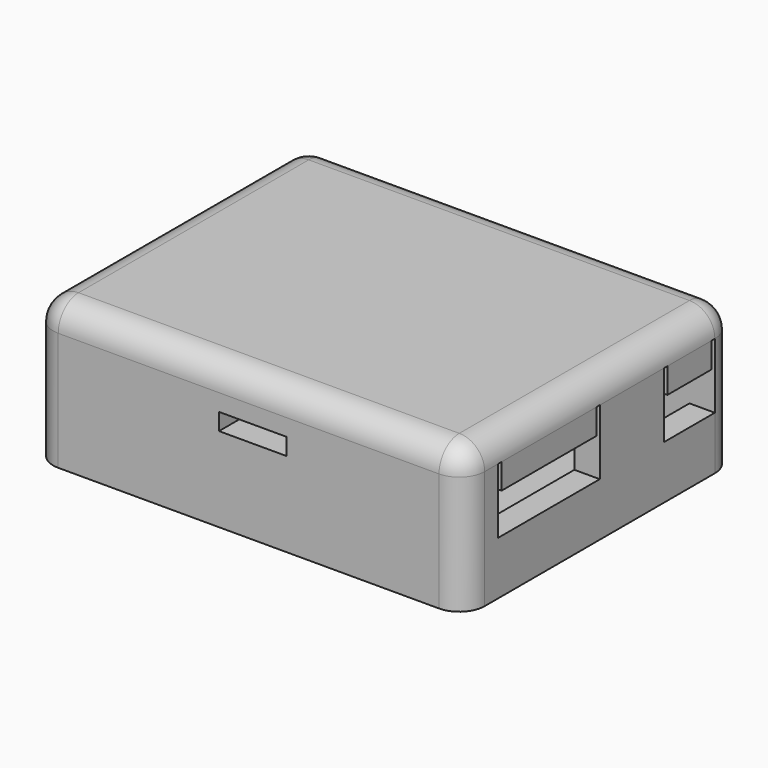
from build123d import *

# Parameters (mm, degrees)
F0_W      = 51
F0_H      = 40
F1_DEPTH  = 14
F2_T      = -3
F3_W      = 7.5
F3_H      = 7.7
F3_W_2    = 15
F4_DEPTH  = 25
F5_W      = 28
F5_H      = 7.7
F6_DEPTH  = 25
F7_W      = 8
F7_H      = 2
F8_DEPTH  = 40.001
F9_R      = 2.99999
F10_W     = 51
F10_H     = 40
F11_DEPTH = 3
F13_DEPTH = 3
F14_W     = 44
F14_H     = 33
F15_DEPTH = 3
F16_R     = 2.99999


# Not quite as in the source:
# - a fillet or chamfer is up to 0.001 mm smaller than in the source, because OpenCascade refuses the exact size


with BuildPart() as f1:
    # F0 (on Top) → F1 (new body)
    with BuildSketch(Plane.XY):
        with Locations((25.5, 20)):
            Rectangle(F0_W, F0_H)
    extrude(amount=F1_DEPTH)

    # F2
    f2_openings = [f1.faces().sort_by_distance(p)[0] for p in [
        (25.5, 20, 14),
    ]]
    offset(amount=F2_T, openings=f2_openings)

    # F3 (on face) → F4 (cut)
    with BuildSketch(Plane.YZ.offset(51)):
        with Locations((33.25, 10.15)):
            Rectangle(F3_W, F3_H)
        with Locations((12.5, 10.15)):
            Rectangle(F3_W_2, F3_H)
    extrude(amount=-F4_DEPTH, mode=Mode.SUBTRACT)

    # F5 (on face) → F6 (cut)
    with BuildSketch(Plane(origin=(0, 0, 0), x_dir=(0, -1, 0), z_dir=(-1, 0, 0))):
        with Locations((-23, 10.15)):
            Rectangle(F5_W, F5_H)
    extrude(amount=-F6_DEPTH, mode=Mode.SUBTRACT)

    # F7 (on face) → F8 (cut, through all)
    with BuildSketch(Plane.XZ):
        with Locations((26, 11)):
            Rectangle(F7_W, F7_H)
    extrude(amount=-F8_DEPTH, mode=Mode.SUBTRACT)

    # F9 (radius 3 in the source; OpenCascade refuses exactly that, so slightly less here)
    f9_edges = [f1.edges().sort_by_distance(p)[0] for p in [
        (0, 0, 7),
        (51, 0, 7),
        (51, 40, 7),
        (0, 40, 7),
    ]]
    fillet(f9_edges, radius=F9_R)


with BuildPart() as f11:
    # F10 (on face) → F11 (new body)
    with BuildSketch(Plane.XY.offset(14)):
        with Locations((25.5, 20)):
            Rectangle(F10_W, F10_H)
    extrude(amount=F11_DEPTH)

    # F12 (on face) → F13 (join)
    with BuildSketch(Plane(origin=(0, 0, 14), x_dir=(1, 0, 0), z_dir=(0, 0, -1))):
        Polygon((0, -36.5), (3.5, -36.5), (47.5, -36.5), (51, -36.5), (51, -30), (47.5, -30), (47.5, -19.5), (51, -19.5), (51, -5.5), (47.5, -5.5), (47.5, -3.5), (3.5, -3.5), (3.5, -9.5), (0, -9.5), align=None)
    extrude(amount=F13_DEPTH)

    # F14 (on face) → F15 (cut)
    with BuildSketch(Plane(origin=(0, 0, 11), x_dir=(1, 0, 0), z_dir=(0, 0, -1))):
        with Locations((25.5, -20)):
            Rectangle(F14_W, F14_H)
    extrude(amount=-F15_DEPTH, mode=Mode.SUBTRACT)

    # F16 (radius 3 in the source; OpenCascade refuses exactly that, so slightly less here)
    f16_edges = [f11.edges().sort_by_distance(p)[0] for p in [
        (0, 40, 15.5),
        (51, 40, 15.5),
        (25.5, 40, 17),
        (51, 20, 17),
        (0, 0, 15.5),
        (0, 20, 17),
        (25.5, 0, 17),
        (51, 0, 15.5),
    ]]
    fillet(f16_edges, radius=F16_R)


solid = Compound([f1.part, f11.part])
